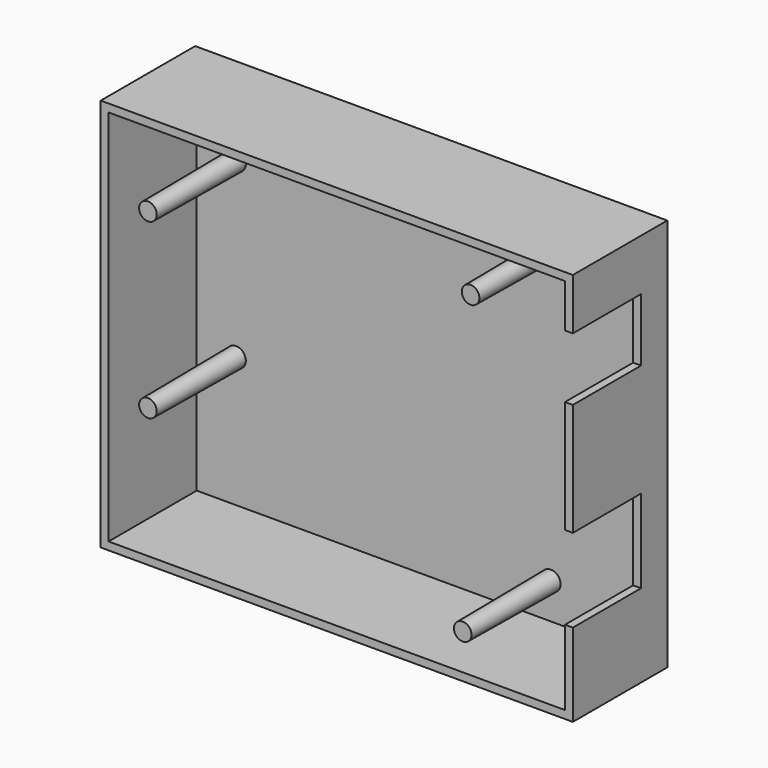
from build123d import *

# Parameters (mm, degrees)
F0_W     = 76.2
F0_H     = 63.5
F1_DEPTH = 19.05
F3_T     = -1.27
F2_R     = 1.5875
F4_DEPTH = 19.05
F4_TAPER = 0.5
F5_W     = 0.22
F5_H     = 10.16
F5_W_2   = 13.75
F5_H_2   = 13.462
F6_DEPTH = 1.27


# Not quite as in the source:
# - a feature names something its author has since deleted; it is built from what else it names


with BuildPart() as f1:
    # F0 (on Front) → F1 (new body)
    with BuildSketch(Plane.XZ):
        with Locations((38.1, 31.75)):
            Rectangle(F0_W, F0_H)
    extrude(amount=F1_DEPTH)

    # F3
    f3_openings = [f1.faces().sort_by_distance(p)[0] for p in [
        (38.1, -19.05, 31.75),
    ]]
    offset(amount=F3_T, openings=f3_openings)

    # F2 (on face) → F4 (join)
    with BuildSketch(Plane.XZ):
        with Locations((59.69, 55.3212)):
            Circle(F2_R)
        with Locations((7.62, 50.2412)):
            Circle(F2_R)
        with Locations((7.62, 22.3012)):
            Circle(F2_R)
        with Locations((58.42, 7.0612)):
            Circle(F2_R)
    extrude(amount=F4_DEPTH, taper=F4_TAPER)

    # F5 (on face) → F6 (cut)
    with BuildSketch(Plane.YZ.offset(76.2)):
        with Locations((-19.16, 50.12)):
            Rectangle(F5_W, F5_H)
        with Locations((-12.175, 50.12)):
            Rectangle(F5_W_2, F5_H)
        with Locations((-19.16, 20.131)):
            Rectangle(F5_W, F5_H_2)
        with Locations((-12.175, 20.131)):
            Rectangle(F5_W_2, F5_H_2)
    extrude(amount=-F6_DEPTH, mode=Mode.SUBTRACT)


solid = f1.part
